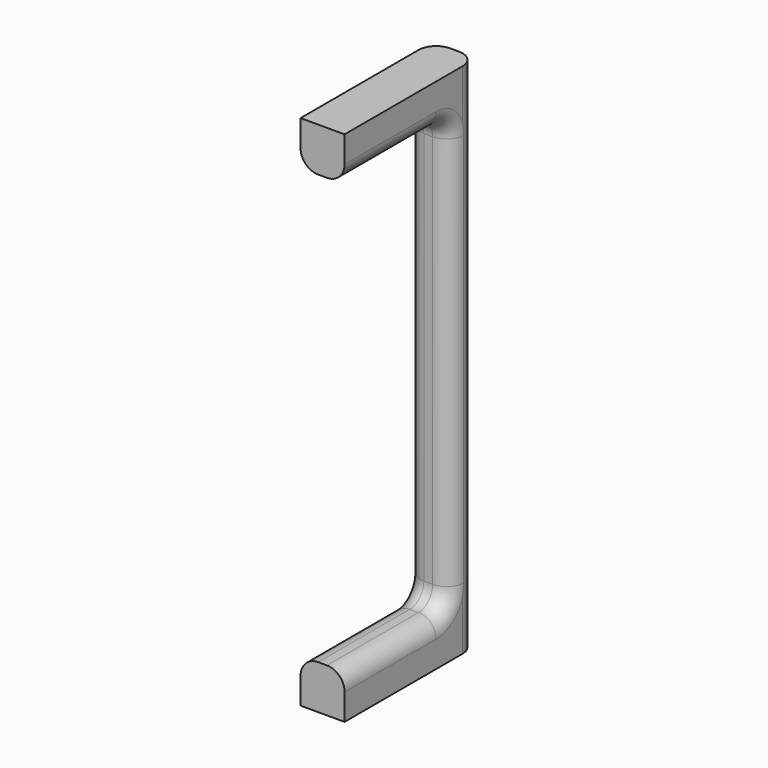
from build123d import *

# Parameters (mm, degrees)
F0_W         = 76.2
F0_H         = 25.4
F1_DEPTH     = 25.4
F2_T1_DEPTH  = 25.4
F2_T3_DEPTH  = 349.25
F2_T5_DEPTH  = 91.44
F2_T7_DEPTH  = 227.33
F2_T10_ANGLE = 90
F2_T12_ANGLE = 90
F2_T14_ANGLE = 90
F2_T16_ANGLE = 90


# Not quite as in the source:
# - a fillet or chamfer that OpenCascade refuses, or shapes differently, is made with other operations: its cross-section is extruded or revolved along the edge and cut away or added


with BuildPart() as f1:
    # F0 (on Right) → F1 (new body)
    with BuildSketch(Plane.YZ):
        Polygon((19.05, 139.6934016338), (0, 139.6934016338), (0, 114.2934016338), (0, 0), (0, -133.3565983662), (-76.2, -133.3565983662), (-76.2, -158.7565983662), (19.05, -158.7565983662), align=None)
        with Locations((-38.1, 126.9934016338)):
            Rectangle(F0_W, F0_H)
    extrude(amount=F1_DEPTH)

    # F2: fillet of radius 10.16 on 10 edges, made by hand

    # F2_s2 → F2_t1 (join)
    with BuildSketch(Plane.YZ):
        with BuildLine():
            ThreePointArc((-10.16, 114.2934016338), (-2.9757951031, 111.3176065306), (0, 104.1334016338))
            Line((0, 104.1334016338), (0, 114.2934016338))
            Line((0, 114.2934016338), (-10.16, 114.2934016338))
        make_face()
        with BuildLine():
            ThreePointArc((0, -123.1965983662), (-2.9757951031, -130.3808032631), (-10.16, -133.3565983662))
            Line((-10.16, -133.3565983662), (0, -133.3565983662))
            Line((0, -133.3565983662), (0, -123.1965983662))
        make_face()
    extrude(amount=F2_T1_DEPTH)

    # F2_s4 → F2_t3 (cut)
    with BuildSketch(Plane.XY.offset(-184.1565983662)):
        with BuildLine():
            ThreePointArc((10.16, 19.05), (2.9757951031, 16.0742048969), (0, 8.89))
            Line((0, 8.89), (0, 19.05))
            Line((0, 19.05), (10.16, 19.05))
        make_face()
        with BuildLine():
            ThreePointArc((15.24, 19.05), (22.4242048969, 16.0742048969), (25.4, 8.89))
            Line((25.4, 8.89), (25.4, 19.05))
            Line((25.4, 19.05), (15.24, 19.05))
        make_face()
    extrude(amount=F2_T3_DEPTH, mode=Mode.SUBTRACT)

    # F2_s6 → F2_t5 (cut)
    with BuildSketch(Plane.XZ.offset(10.16)):
        with BuildLine():
            ThreePointArc((25.4, 124.4534016338), (22.4242048969, 117.2691967369), (15.24, 114.2934016338))
            Line((15.24, 114.2934016338), (25.4, 114.2934016338))
            Line((25.4, 114.2934016338), (25.4, 124.4534016338))
        make_face()
        with BuildLine():
            ThreePointArc((25.4, -143.5165983662), (22.4242048969, -136.3323934694), (15.24, -133.3565983662))
            Line((15.24, -133.3565983662), (25.4, -133.3565983662))
            Line((25.4, -133.3565983662), (25.4, -143.5165983662))
        make_face()
        with BuildLine():
            ThreePointArc((0, -143.5165983662), (2.9757951031, -136.3323934694), (10.16, -133.3565983662))
            Line((10.16, -133.3565983662), (0, -133.3565983662))
            Line((0, -133.3565983662), (0, -143.5165983662))
        make_face()
        with BuildLine():
            ThreePointArc((0, 124.4534016338), (2.9757951031, 117.2691967369), (10.16, 114.2934016338))
            Line((10.16, 114.2934016338), (0, 114.2934016338))
            Line((0, 114.2934016338), (0, 124.4534016338))
        make_face()
    extrude(amount=F2_T5_DEPTH, mode=Mode.SUBTRACT)

    # F2_s8 → F2_t7 (cut)
    with BuildSketch(Plane.XY.offset(-123.1965983662)):
        with BuildLine():
            ThreePointArc((25.4, 10.16), (22.4242048969, 2.9757951031), (15.24, 0))
            Line((15.24, 0), (25.4, 0))
            Line((25.4, 0), (25.4, 10.16))
        make_face()
        with BuildLine():
            ThreePointArc((0, 10.16), (2.9757951031, 2.9757951031), (10.16, 0))
            Line((10.16, 0), (0, 0))
            Line((0, 0), (0, 10.16))
        make_face()
    extrude(amount=F2_T7_DEPTH, mode=Mode.SUBTRACT)

    # F2_s9 → F2_t10 (revolve, cut)
    with BuildSketch(Plane.XZ.offset(10.16)):
        with BuildLine():
            ThreePointArc((0, 124.4534016338), (2.9757951031, 117.2691967369), (10.16, 114.2934016338))
            Line((10.16, 114.2934016338), (0, 114.2934016338))
            Line((0, 114.2934016338), (0, 124.4534016338))
        make_face()
    revolve(axis=Axis((0, -10.16, 104.1334016338), (-1, 0, 0)), revolution_arc=F2_T10_ANGLE, mode=Mode.SUBTRACT)

    # F2_s11 → F2_t12 (revolve, cut)
    with BuildSketch(Plane.XY.offset(-123.1965983662)):
        with BuildLine():
            ThreePointArc((0, 10.16), (2.9757951031, 2.9757951031), (10.16, 0))
            Line((10.16, 0), (0, 0))
            Line((0, 0), (0, 10.16))
        make_face()
    revolve(axis=Axis((0, -10.16, -123.1965983662), (-1, 0, 0)), revolution_arc=F2_T12_ANGLE, mode=Mode.SUBTRACT)

    # F2_s13 → F2_t14 (revolve, cut)
    with BuildSketch(Plane.XY.offset(-123.1965983662)):
        with BuildLine():
            ThreePointArc((25.4, 10.16), (22.4242048969, 2.9757951031), (15.24, 0))
            Line((15.24, 0), (25.4, 0))
            Line((25.4, 0), (25.4, 10.16))
        make_face()
    revolve(axis=Axis((25.4, -10.16, -123.1965983662), (-1, 0, 0)), revolution_arc=F2_T14_ANGLE, mode=Mode.SUBTRACT)

    # F2_s15 → F2_t16 (revolve, cut)
    with BuildSketch(Plane.XZ.offset(10.16)):
        with BuildLine():
            ThreePointArc((25.4, 124.4534016338), (22.4242048969, 117.2691967369), (15.24, 114.2934016338))
            Line((15.24, 114.2934016338), (25.4, 114.2934016338))
            Line((25.4, 114.2934016338), (25.4, 124.4534016338))
        make_face()
    revolve(axis=Axis((25.4, -10.16, 104.1334016338), (-1, 0, 0)), revolution_arc=F2_T16_ANGLE, mode=Mode.SUBTRACT)


solid = f1.part
